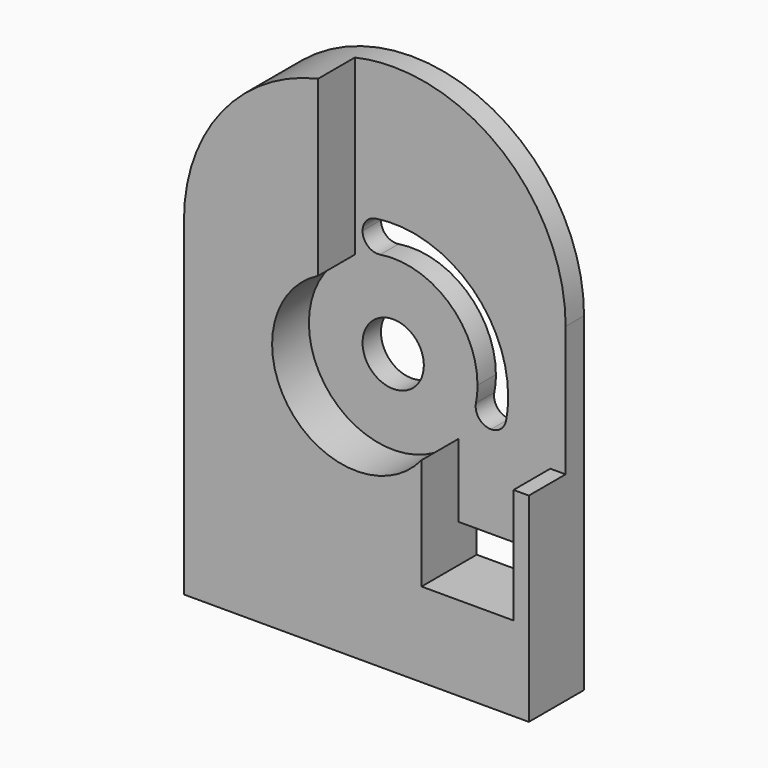
from build123d import *

# Parameters (mm, degrees)
F1_DEPTH  = 9
F3_DEPTH  = 6
F4_R      = 4
F5_DEPTH  = 25
F6_R      = 1.99999
F7_W      = 12
F7_H      = 6
F8_DEPTH  = 15
F9_W      = 12
F9_H      = 5
F10_DEPTH = 25


# Not quite as in the source:
# - a fillet or chamfer is up to 0.001 mm smaller than in the source, because OpenCascade refuses the exact size


with BuildPart() as f1:
    # F0 (on Front) → F1 (new body)
    with BuildSketch(Plane.XZ):
        with BuildLine():
            ThreePointArc((0, 44), (-15.9099025767, 37.4099025767), (-22.5, 21.5))
            Line((-22.5, 21.5), (0, 21.5))
            Line((0, 21.5), (0, 44))
        make_face()
        with BuildLine():
            ThreePointArc((0, -1), (-15.9099025767, 5.5900974233), (-22.5, 21.5))
            Line((-22.5, 21.5), (-22.5, -21.5))
            Line((-22.5, -21.5), (0, -21.5))
            Line((0, -21.5), (0, -1))
        make_face()
        with BuildLine():
            Line((0, 21.5), (-22.5, 21.5))
            ThreePointArc((-22.5, 21.5), (-15.9099025767, 5.5900974233), (0, -1))
            Line((0, -1), (0, 21.5))
        make_face()
        with BuildLine():
            Line((0, 44), (0, 21.5))
            Line((0, 21.5), (22.5, 21.5))
            ThreePointArc((22.5, 21.5), (15.9099025767, 37.4099025767), (0, 44))
        make_face()
        with BuildLine():
            Line((22.5, 21.5), (0, 21.5))
            Line((0, 21.5), (0, -1))
            ThreePointArc((0, -1), (15.9099025767, 5.5900974233), (22.5, 21.5))
        make_face()
        with BuildLine():
            ThreePointArc((22.5, 21.5), (15.9099025767, 5.5900974233), (0, -1))
            Line((0, -1), (0, -21.5))
            Line((0, -21.5), (22.5, -21.5))
            Line((22.5, -21.5), (22.5, 21.5))
        make_face()
    extrude(amount=F1_DEPTH)

    # F2 (on face) → F3 (cut)
    with BuildSketch(Plane.XZ.offset(9)):
        with BuildLine():
            Line((0, 30.8210086077), (0, 44))
            ThreePointArc((0, 44), (-2.5157755473, 43.8589103803), (-5, 43.4374109685))
            Line((-5, 43.4374109685), (-5, 30.8210086077))
            Line((-5, 30.8210086077), (0, 30.8210086077))
        make_face()
        with BuildLine():
            Line((0, 22), (0, 30.8210086077))
            Line((0, 30.8210086077), (-5, 30.8210086077))
            Line((-5, 30.8210086077), (-5, 20.7979589711))
            ThreePointArc((-5, 20.7979589711), (-2.5712303784, 21.695268783), (0, 22))
        make_face()
        with BuildLine():
            ThreePointArc((11, 11), (7.7781745931, 18.7781745931), (0, 22))
            ThreePointArc((0, 22), (-2.5712303784, 21.695268783), (-5, 20.7979589711))
            ThreePointArc((-5, 20.7979589711), (-8.3760412767, 3.8696470964), (8.8741196746, 4.5))
            ThreePointArc((8.8741196746, 4.5), (10.4550302826, 7.5805933571), (11, 11))
        make_face()
        with BuildLine():
            ThreePointArc((22.5, 21.5), (15.9099025767, 37.4099025767), (0, 44))
            Line((0, 44), (0, 30.8210086077))
            Line((0, 30.8210086077), (0, 22))
            ThreePointArc((0, 22), (7.7781745931, 18.7781745931), (11, 11))
            ThreePointArc((11, 11), (10.4550302826, 7.5805933571), (8.8741196746, 4.5))
            Line((8.8741196746, 4.5), (22.5, 4.5))
            Line((22.5, 4.5), (22.5, 21.5))
        make_face()
    extrude(amount=-F3_DEPTH, mode=Mode.SUBTRACT)

    # F4 (on face) → F5 (cut)
    with BuildSketch(Plane.XZ.offset(3)):
        with BuildLine():
            ThreePointArc((-4, 21.246950766), (6.204836823, 20.0829510623), (11, 11))
            ThreePointArc((11, 11), (10.7566660599, 8.6991012027), (10.0374299499, 6.5))
            Line((10.0374299499, 6.5), (14.3090880213, 6.5))
            ThreePointArc((14.3090880213, 6.5), (14.8262658872, 8.7236345108), (15, 11))
            ThreePointArc((15, 11), (9.0829510623, 22.9373363863), (-4, 25.4568322948))
            Line((-4, 25.4568322948), (-4, 21.246950766))
        make_face()
        with Locations((0, 11)):
            Circle(F4_R)
    extrude(amount=-F5_DEPTH, mode=Mode.SUBTRACT)

    # F6 (radius 2 in the source; OpenCascade refuses exactly that, so slightly less here)
    f6_edges = [f1.edges().sort_by_distance(p)[0] for p in [
        (-4, -1.5, 25.456832),
        (-4, -1.5, 21.246951),
        (14.309088, -1.5, 6.5),
        (10.03743, -1.5, 6.5),
    ]]
    fillet(f6_edges, radius=F6_R)

    # F7 (on face) → F8 (cut)
    with BuildSketch(Plane.XY.offset(4.5)):
        with Locations((14.5, -6)):
            Rectangle(F7_W, F7_H)
    extrude(amount=-F8_DEPTH, mode=Mode.SUBTRACT)

    # F9 (on face) → F10 (cut)
    with BuildSketch(Plane.XZ.offset(3)):
        with Locations((14.5, -8)):
            Rectangle(F9_W, F9_H)
    extrude(amount=-F10_DEPTH, mode=Mode.SUBTRACT)


solid = f1.part
